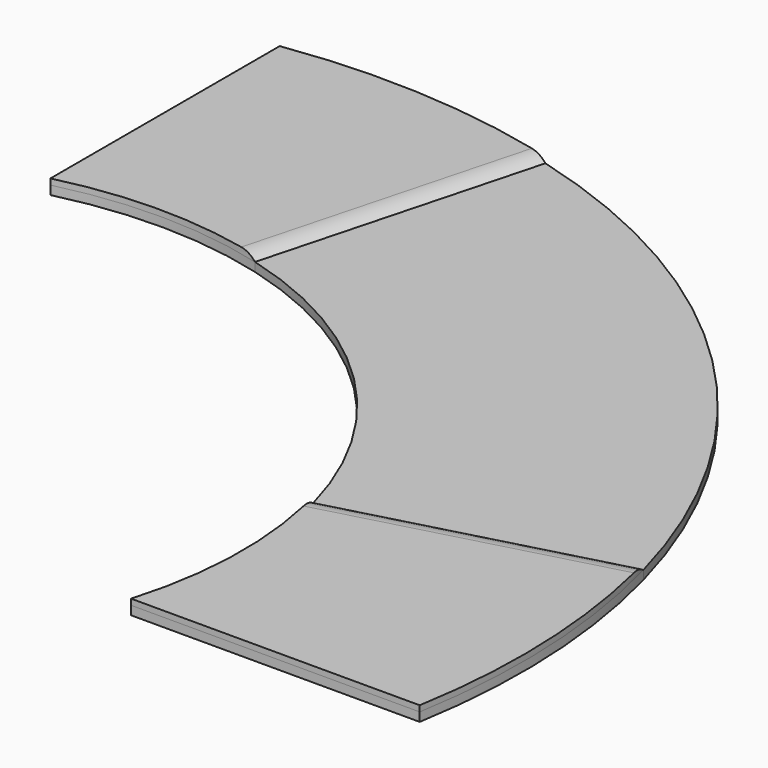
from build123d import *

# Parameters (mm, degrees)
F1_DEPTH      = 1
F2_DEPTH      = 1.5
F3_SIZE       = 0.99999
F3_2_SIZE     = 0.99999
F4_T1_DEPTH   = 58.00296827
F4_2_T1_DEPTH = 58.00296827


# Not quite as in the source:
# - a fillet or chamfer that OpenCascade refuses, or shapes differently, is made with other operations: its cross-section is extruded or revolved along the edge and cut away or added
# - a fillet or chamfer is up to 0.001 mm smaller than in the source, because OpenCascade refuses the exact size


with BuildPart() as f1:
    # F0 (on Top) → F1 (new body)
    with BuildSketch(Plane.XY):
        with BuildLine():
            ThreePointArc((-17, 67.9043444855), (0.5771188901, 69.9976209152), (18.1173331572, 67.6148078402))
            Line((18.1173331572, 67.6148078402), (30.5406678037, 113.9793239405))
            ThreePointArc((30.5406678037, 113.9793239405), (6.9125327944, 117.7974344635), (-17, 116.7690827053))
            Line((-17, 116.7690827053), (-17, 67.9043444855))
        make_face()
    extrude(amount=F1_DEPTH)

    # F3 (size 1 in the source; OpenCascade refuses exactly that, so slightly less here)
    f3_edges = [f1.edges().sort_by_distance(p)[0] for p in [
        (24.329, 90.797066, 1),
    ]]
    chamfer(f3_edges, length=F3_SIZE)

    # F4: fillet of radius 5 on 1 edges, made by hand

    # F4_s2 → F4_t1 (cut)
    with BuildSketch(Plane(origin=(16.8213913237, 62.778287074, 0), x_dir=(0, 0, 1), z_dir=(0.2588190451, 0.9659258263, 0))):
        with BuildLine():
            ThreePointArc((1e-05, 0), (0.7434191255, -1.4188557423), (1, -2.9999866666))
            Line((1, -2.9999866666), (1, -0.99999))
            Line((1, -0.99999), (1e-05, 0))
        make_face()
    extrude(amount=F4_T1_DEPTH, mode=Mode.SUBTRACT)


with BuildPart() as f1b:
    # F0 (on Top) → F1, piece 2 (new body)
    with BuildSketch(Plane.XY):
        with BuildLine():
            ThreePointArc((67.6148078402, 18.1173331572), (69.9931634577, -0.9782991276), (67.082039325, -20))
            Line((67.082039325, -20), (116.2928143774, -20))
            ThreePointArc((116.2928143774, -20), (117.8766482255, 5.3957834406), (113.9793239405, 30.5406678037))
            Line((113.9793239405, 30.5406678037), (67.6148078402, 18.1173331572))
        make_face()
    extrude(amount=F1_DEPTH)

    # F3#2 (size 1 in the source; OpenCascade refuses exactly that, so slightly less here)
    f3_2_edges = [f1b.edges().sort_by_distance(p)[0] for p in [
        (90.797066, 24.329, 1),
    ]]
    chamfer(f3_2_edges, length=F3_2_SIZE)

    # F4#2: fillet of radius 5 on 1 edges, made by hand

    # F4_2_s2 → F4_2_t1 (cut)
    with BuildSketch(Plane(origin=(118.8048521275, 31.8336641845, 0), x_dir=(0, 0, 1), z_dir=(-0.9659258263, -0.2588190451, 0))):
        with BuildLine():
            ThreePointArc((1e-05, 0), (0.7434191255, -1.4188557423), (1, -2.9999866666))
            Line((1, -2.9999866666), (1, -0.99999))
            Line((1, -0.99999), (1e-05, 0))
        make_face()
    extrude(amount=F4_2_T1_DEPTH, mode=Mode.SUBTRACT)


with BuildPart() as f2:
    # F0 (on Top) → F2 (new body)
    with BuildSketch(Plane.XY):
        with BuildLine():
            ThreePointArc((-17, 67.9043444855), (0.5771188901, 69.9976209152), (18.1173331572, 67.6148078402))
            Line((18.1173331572, 67.6148078402), (30.5406678037, 113.9793239405))
            ThreePointArc((30.5406678037, 113.9793239405), (6.9125327944, 117.7974344635), (-17, 116.7690827053))
            Line((-17, 116.7690827053), (-17, 67.9043444855))
        make_face()
        with BuildLine():
            ThreePointArc((18.1173331572, 67.6148078402), (49.4974746831, 49.4974746831), (67.6148078402, 18.1173331572))
            Line((67.6148078402, 18.1173331572), (113.9793239405, 30.5406678037))
            ThreePointArc((113.9793239405, 30.5406678037), (83.4386561368, 83.4386561368), (30.5406678037, 113.9793239405))
            Line((30.5406678037, 113.9793239405), (18.1173331572, 67.6148078402))
        make_face()
        with BuildLine():
            ThreePointArc((67.6148078402, 18.1173331572), (69.9931634577, -0.9782991276), (67.082039325, -20))
            Line((67.082039325, -20), (116.2928143774, -20))
            ThreePointArc((116.2928143774, -20), (117.8766482255, 5.3957834406), (113.9793239405, 30.5406678037))
            Line((113.9793239405, 30.5406678037), (67.6148078402, 18.1173331572))
        make_face()
    extrude(amount=-F2_DEPTH)


solid = Compound([f1.part, f1b.part, f2.part])
